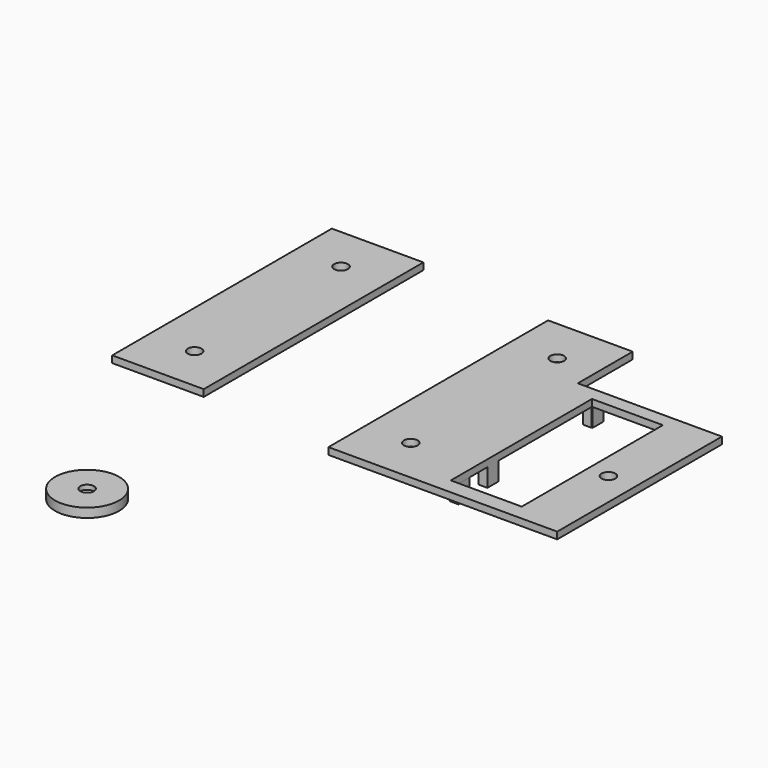
from build123d import *

# Parameters (mm, degrees)
F1_W      = 20
F1_H      = 60
F1_R      = 1.5
F2_DEPTH  = 1.5
F0_R      = 1.5
F0_W      = 15.5
F0_H      = 38.5640101805
F3_DEPTH  = 1.5
F4_W      = 2
F4_H      = 3
F5_DEPTH  = 4
F6_R      = 4
F6_R_2    = 1.5
F7_DEPTH  = 1
F9_DEPTH  = 1
F6_R_3    = 7
F10_DEPTH = 2


# Not quite as in the source:
# - a feature names something its author has since deleted; it is built from what else it names


with BuildPart() as f2:
    # F1 (on Top) → F2 (new body)
    with BuildSketch(Plane.XY):
        with Locations((-50, 30)):
            Rectangle(F1_W, F1_H)
        with Locations((-50, 10)):
            Circle(F1_R, mode=Mode.SUBTRACT)
        with Locations((-50, 50)):
            Circle(F1_R, mode=Mode.SUBTRACT)
    extrude(amount=F2_DEPTH)


with BuildPart() as f3:
    # F0 (on Top) → F3 (new body)
    with BuildSketch(Plane.XY):
        Polygon((-10, 56.5640101805), (-10, -3.4359898195), (40, -3.4359898195), (40, 41.5640101805), (8.5, 41.5640101805), (8.5, 56.5640101805), align=None)
        with Locations((0, 6.5640101805)):
            Circle(F0_R, mode=Mode.SUBTRACT)
        with Locations((21.75, 19.2820050903)):
            Rectangle(F0_W, F0_H, mode=Mode.SUBTRACT)
        with Locations((34, 18.0640101805)):
            Circle(F0_R, mode=Mode.SUBTRACT)
        with Locations((0, 46.5640101805)):
            Circle(F0_R, mode=Mode.SUBTRACT)
    extrude(amount=F3_DEPTH)

    # F4 (on face) → F5 (join)
    with BuildSketch(Plane.XY):
        with Locations((13, 11.5)):
            Rectangle(F4_W, F4_H)
        with Locations((12.9658896476, 3.6489479244)):
            Rectangle(F4_W, F4_H)
        Polygon((12.1644257344, 38.4399581365), (14, 38.4399581365), (14, 38.5640101805), (14.1644257344, 38.5640101805), (14.1644257344, 41.4399581365), (12.1644257344, 41.4399581365), align=None)
    extrude(amount=-F5_DEPTH)


with BuildPart() as f7:
    # F6 (on Top) → F7 (new body)
    with BuildSketch(Plane.XY):
        with Locations((-34.3638770282, -38.9125682414)):
            Circle(F6_R)
        with Locations((-34.3638770282, -38.9125682414)):
            Circle(F6_R_2, mode=Mode.SUBTRACT)
    extrude(amount=-F7_DEPTH)


with BuildPart() as f9:
    # F6 (on Top) → F9 (new body)
    with BuildSketch(Plane.XY):
        with Locations((-34.3638770282, -38.9125682414)):
            Circle(F6_R)
        with Locations((-34.3638770282, -38.9125682414)):
            Circle(F6_R_2, mode=Mode.SUBTRACT)
    extrude(amount=-F9_DEPTH)

    # F6 (on Top) → F10 (join)
    with BuildSketch(Plane.XY):
        with Locations((-34.3638770282, -38.9125682414)):
            Circle(F6_R_3)
        with Locations((-34.3638770282, -38.9125682414)):
            Circle(F6_R, mode=Mode.SUBTRACT)
    extrude(amount=-F10_DEPTH)


solid = Compound([f2.part, f3.part, f9.part])
